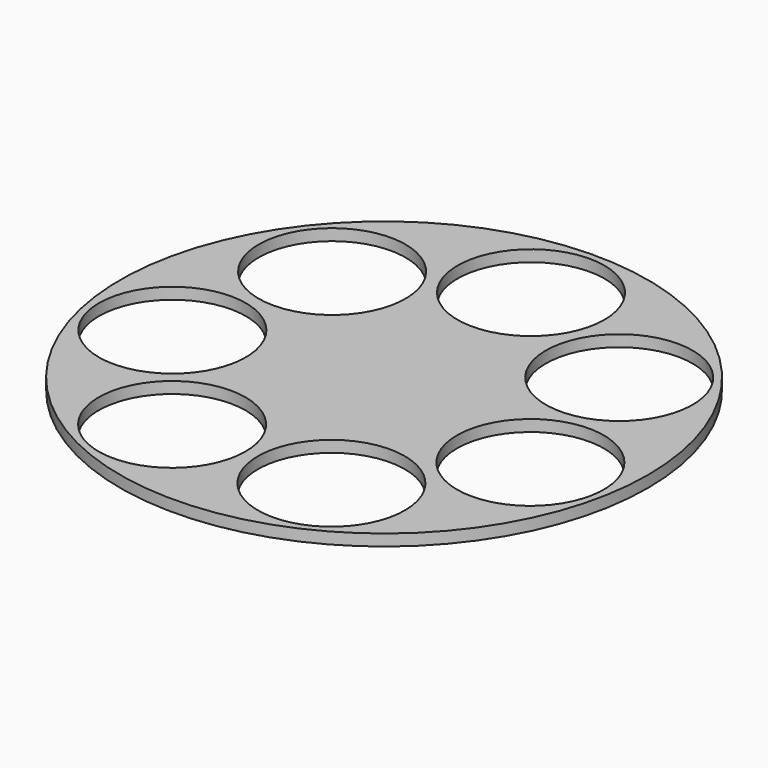
from build123d import *

# Parameters (mm, degrees)
F0_R            = 115
F1_DEPTH        = 5
F2_R            = 32
F3_DEPTH        = 5
F3_COPIES_COUNT = 7


# Not quite as in the source:
# - a pattern or mirror of a feature is missing from the dataset's text; its kind, count and spacing are read off the source's solid


with BuildPart() as f1:
    # F0 (on Top) → F1 (new body)
    with BuildSketch(Plane.XY):
        Circle(F0_R)
    extrude(amount=F1_DEPTH)

    # F2 (on face) → F3 (cut)
    with BuildSketch(Plane.XY.offset(5)):
        with Locations((0, 80)):
            Circle(F2_R)
    f3 = extrude(amount=-F3_DEPTH, mode=Mode.SUBTRACT)

    # F3_copies: F3 ×7 about axis
    f3_copies_axis = Axis((0, 0, 0), (0, 0, 1))
    for i in range(1, F3_COPIES_COUNT):
        add(f3.rotate(f3_copies_axis, i * 360 / F3_COPIES_COUNT), mode=Mode.SUBTRACT)


solid = f1.part
